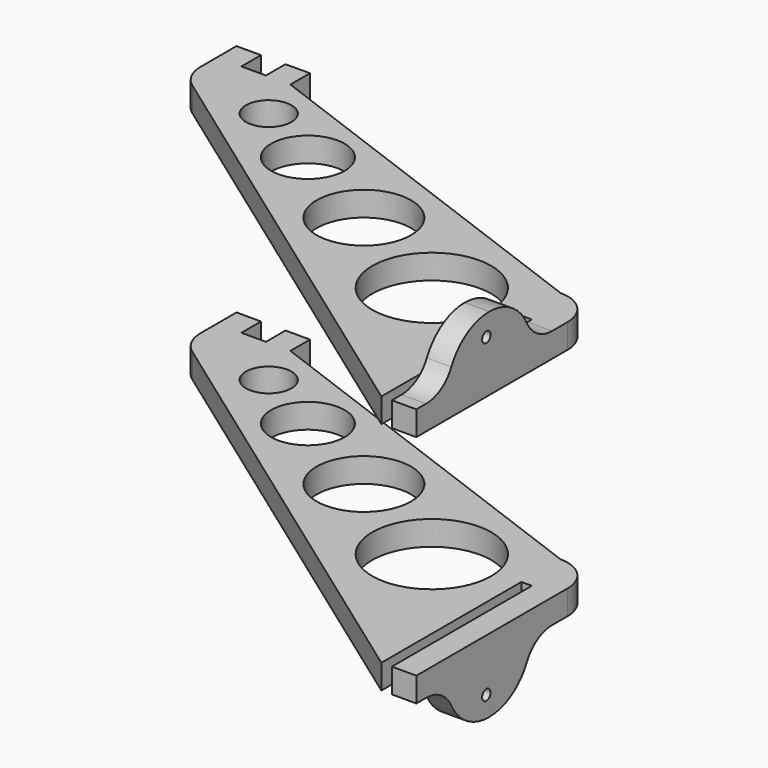
from build123d import *

# Parameters (mm, degrees)
F2_DEPTH    = 7
F1_R        = 17
F1_R_2      = 13.5
F1_R_3      = 10.5
F1_R_4      = 6.5
F3_DEPTH    = 25
F4_W        = 30
F4_H        = 14
F5_DEPTH    = 7
F7_T1_DEPTH = 81.8331477355
F8_R        = 10
F6_R        = 1.5
F9_DEPTH    = 25
F10_R       = 9.99999
F11_R       = 10


# Not quite as in the source:
# - a fillet or chamfer that OpenCascade refuses, or shapes differently, is made with other operations: its cross-section is extruded or revolved along the edge and cut away or added
# - a fillet or chamfer is up to 0.001 mm smaller than in the source, because OpenCascade refuses the exact size


with BuildPart() as f2:
    # F0 (on Top) → F2 (new body)
    with BuildSketch(Plane.XY):
        Polygon((-7, 0), (0, 0), (0, 64), (-10, 64), (-120, 105), (-120, 112), (-127, 112), (-127, 105), (-134, 105), (-134, 112), (-141, 112), (-141, 94), (-10, 0), (-10, 50), (-7, 50), align=None)
    extrude(amount=F2_DEPTH)

    # F1 (on Top) → F3 (cut)
    with BuildSketch(Plane.XY):
        with Locations((-34, 48)):
            Circle(F1_R)
        with Locations((-67, 65)):
            Circle(F1_R_2)
        with Locations((-95, 80)):
            Circle(F1_R_3)
        with Locations((-115, 91)):
            Circle(F1_R_4)
    extrude(amount=F3_DEPTH, mode=Mode.SUBTRACT)

    # F4 (on face) → F5 (join)
    with BuildSketch(Plane.YZ):
        with Locations((25.9959850088, 14)):
            Rectangle(F4_W, F4_H)
    extrude(amount=-F5_DEPTH)

    # F7: fillet of radius 15 on 2 edges, made by hand

    # F7_s2 → F7_t1 (cut)
    with BuildSketch(Plane.YZ.offset(-44.4165738677)):
        with BuildLine():
            ThreePointArc((10.9959850088, 7), (15.7156637899, 16.9544511501), (25.9626145559, 21))
            Line((25.9626145559, 21), (10.9959850088, 21))
            Line((10.9959850088, 21), (10.9959850088, 7))
        make_face()
        with BuildLine():
            ThreePointArc((40.9959850088, 7), (36.2763062276, 16.9544511501), (26.0293554617, 21))
            Line((26.0293554617, 21), (40.9959850088, 21))
            Line((40.9959850088, 21), (40.9959850088, 7))
        make_face()
    extrude(amount=F7_T1_DEPTH, mode=Mode.SUBTRACT)

    # F8
    f8_edges = [f2.edges().sort_by_distance(p)[0] for p in [
        (-3.5, 10.995985, 7),
        (-3.5, 40.995985, 7),
    ]]
    fillet(f8_edges, radius=F8_R)

    # F6 (on face) → F9 (cut)
    with BuildSketch(Plane.YZ):
        with Locations((24.9959850088, 15)):
            Circle(F6_R)
    extrude(amount=-F9_DEPTH, mode=Mode.SUBTRACT)

    # F10 (radius 10 in the source; OpenCascade refuses exactly that, so slightly less here)
    f10_edges = [f2.edges().sort_by_distance(p)[0] for p in [
        (0, 64, 3.5),
    ]]
    fillet(f10_edges, radius=F10_R)

    # F11
    f11_edges = [f2.edges().sort_by_distance(p)[0] for p in [
        (-141, 94, 3.5),
    ]]
    fillet(f11_edges, radius=F11_R)


with BuildPart() as f12_1:
    # F12: instance of F2
    add(f2.part.mirror(Plane.XY))


with BuildPart() as f12_1_1:
    # F13: moved
    add(f12_1.part.moved(Location((0, 0, -60))))


solid = Compound([f2.part, f12_1_1.part])
